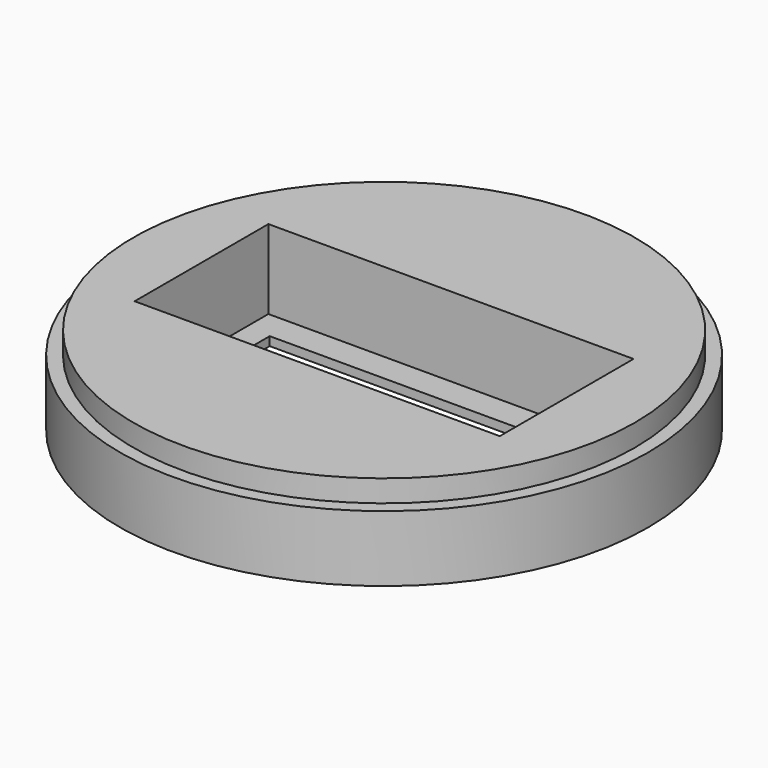
from build123d import *

# Parameters (mm, degrees)
F0_R           = 60
F0_R_2         = 57
F2_DEPTH       = 15
F1_R           = 57
F1_R_2         = 54
F3_DEPTH       = 20
F4_R           = 57
F5_DEPTH       = 10
F7_R           = 54
F8_DEPTH       = 40
F9_W           = 15
F9_H           = 10
F10_DEPTH      = 279.5
F11_DEPTH      = 71.5
F13_R          = 60
F14_DEPTH      = 20
F15_W          = 72
F15_H          = 25
F16_DEPTH      = 20
F17_W          = 83
F17_H          = 38
F18_DEPTH      = 13
F18_DEPTH_BACK = 5
F19_R          = 60
F19_R_2        = 57
F20_DEPTH      = 5


# Not quite as in the source:
# - a feature names something its author has since deleted; it is built from what else it names


with BuildPart() as f2:
    # F0 (on Top) → F2 (new body)
    with BuildSketch(Plane.XY):
        Circle(F0_R)
        Circle(F0_R_2, mode=Mode.SUBTRACT)
    extrude(amount=F2_DEPTH)

    # F1 (on Top) → F3 (join)
    with BuildSketch(Plane.XY):
        Circle(F1_R)
        Circle(F1_R_2, mode=Mode.SUBTRACT)
    extrude(amount=F3_DEPTH)

    # F4 (on Top) → F5 (join)
    with BuildSketch(Plane.XY):
        Circle(F4_R)
    extrude(amount=F5_DEPTH)

    # F7 (on offset) → F8 (cut)
    with BuildSketch(Plane.XY.offset(45)):
        Circle(F7_R)
    extrude(amount=-F8_DEPTH, mode=Mode.SUBTRACT)

    # F9 (on Right) → F10 (cut)
    with BuildSketch(Plane.YZ):
        with Locations((32.5, 60)):
            Rectangle(F9_W, F9_H)
    extrude(amount=F10_DEPTH, mode=Mode.SUBTRACT)

    # F1 (on Top) → F11 (cut)
    with BuildSketch(Plane.XY):
        Circle(F1_R_2)
    extrude(amount=F11_DEPTH, mode=Mode.SUBTRACT)

    # F13 (on Top) → F14 (join)
    with BuildSketch(Plane.XY):
        Circle(F13_R)
    extrude(amount=F14_DEPTH)

    # F15 (on Top) → F16 (cut)
    with BuildSketch(Plane.XY):
        Rectangle(F15_W, F15_H)
    extrude(amount=F16_DEPTH, mode=Mode.SUBTRACT)

    # F17 (on offset) → F18 (cut, two sides)
    with BuildSketch(Plane.XY.offset(15)) as f18_sk:
        Rectangle(F17_W, F17_H)
    extrude(amount=-F18_DEPTH, mode=Mode.SUBTRACT)
    extrude(f18_sk.sketch, amount=F18_DEPTH_BACK, mode=Mode.SUBTRACT)

    # F19 (on face) → F20 (cut)
    with BuildSketch(Plane.XY.offset(20)):
        Circle(F19_R)
        Circle(F19_R_2, mode=Mode.SUBTRACT)
    extrude(amount=-F20_DEPTH, mode=Mode.SUBTRACT)


solid = f2.part
